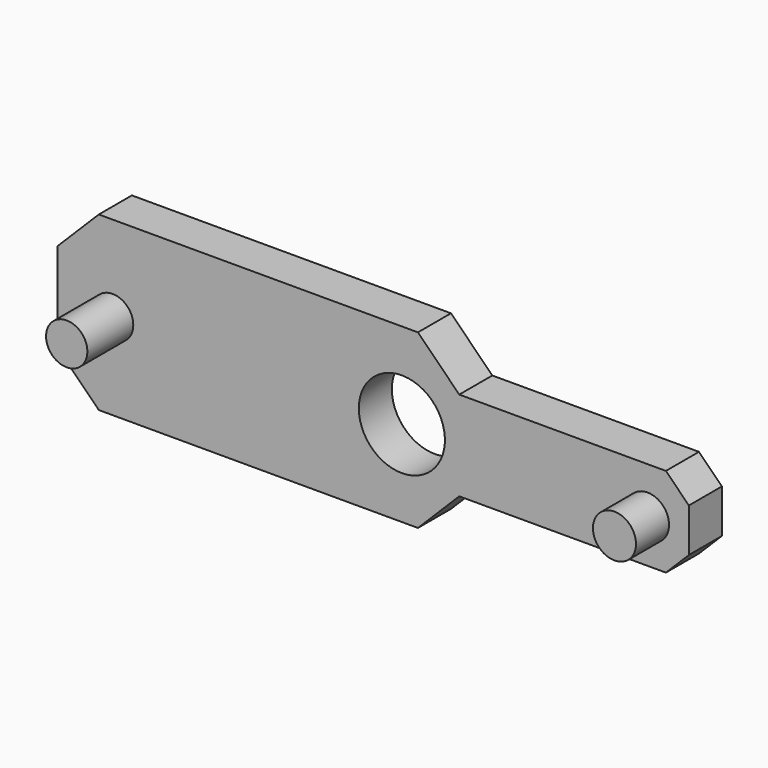
from build123d import *

# Parameters (mm, degrees)
F0_W        = 88.9
F0_H        = 38.1
F1_DEPTH    = 9.144
F2_R        = 4.572
F3_DEPTH    = 12.7
F4_R        = 9.525
F5_DEPTH    = 21.845
F6_SIZE     = 9.144
F7_W        = 9.144
F7_H        = 19.812
F8_DEPTH    = 50.8
F9_T1_DEPTH = 35.2722991577
F10_R       = 4.7625
F11_DEPTH   = 9.144


# Not quite as in the source:
# - a fillet or chamfer that OpenCascade refuses, or shapes differently, is made with other operations: its cross-section is extruded or revolved along the edge and cut away or added


with BuildPart() as f1:
    # F0 (on Front) → F1 (new body)
    with BuildSketch(Plane.XZ):
        with Locations((44.45, 19.05)):
            Rectangle(F0_W, F0_H)
    extrude(amount=F1_DEPTH)

    # F2 (on face) → F3 (join)
    with BuildSketch(Plane.XZ.offset(9.144)):
        with Locations((12.2043658048, 19.05)):
            Circle(F2_R)
    extrude(amount=F3_DEPTH)

    # F4 (on face) → F5 (cut, through all)
    with BuildSketch(Plane(origin=(0, 0, 0), x_dir=(-1, 0, 0), z_dir=(0, 1, 0))):
        with Locations((-76.2, 19.05)):
            Circle(F4_R)
    extrude(amount=-F5_DEPTH, mode=Mode.SUBTRACT)

    # F6
    f6_edges = [f1.edges().sort_by_distance(p)[0] for p in [
        (0, -4.572, 38.1),
        (88.9, -4.572, 38.1),
        (0, -4.572, 0),
        (88.9, -4.572, 0),
    ]]
    chamfer(f6_edges, length=F6_SIZE)

    # F7 (on face) → F8 (join)
    with BuildSketch(Plane.YZ.offset(88.9)):
        with Locations((-4.572, 19.05)):
            Rectangle(F7_W, F7_H)
    extrude(amount=F8_DEPTH)

    # F9: chamfer of 5.08 on 4 edges, made by hand

    # F9_s2 → F9_t1 (cut)
    with BuildSketch(Plane.XZ.offset(-13.0641495789)):
        Polygon((134.62, 28.956), (139.7, 23.876), (139.7, 28.956), align=None)
        Polygon((134.62, 9.144), (139.7, 14.224), (139.7, 9.144), align=None)
    extrude(amount=F9_T1_DEPTH, mode=Mode.SUBTRACT)

    # F10 (on face) → F11 (join)
    with BuildSketch(Plane.XZ.offset(9.144)):
        with Locations((130.556, 18.669)):
            Circle(F10_R)
    extrude(amount=F11_DEPTH)


solid = f1.part
